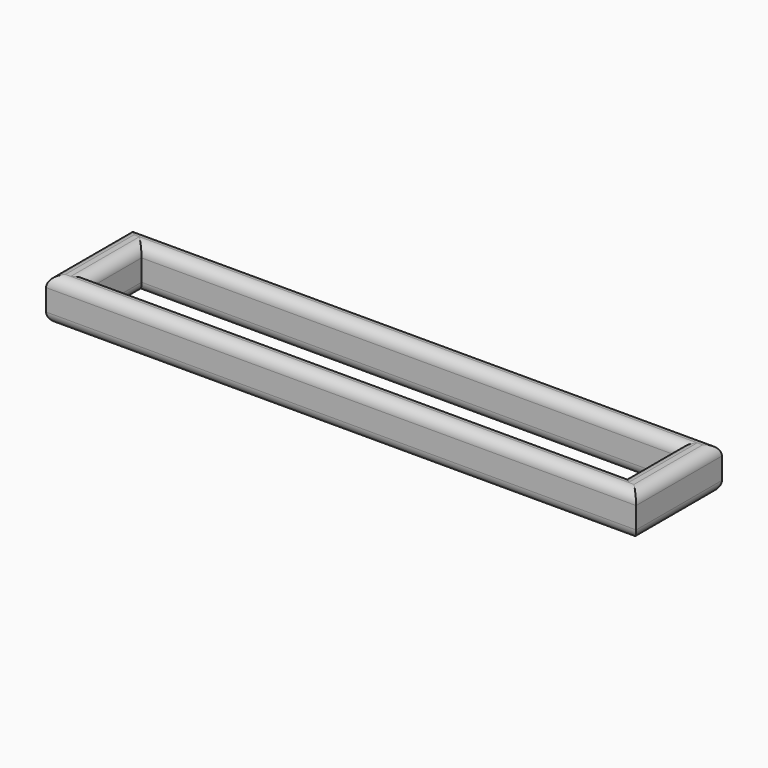
from build123d import *

# Parameters (mm, degrees)
F0_W     = 69.85
F0_H     = 12.7
F0_W_2   = 63.5
F0_H_2   = 7.62
F1_DEPTH = 5.08
F2_R     = 1.26999


# Not quite as in the source:
# - a fillet or chamfer is up to 0.001 mm smaller than in the source, because OpenCascade refuses the exact size


with BuildPart() as f1:
    # F0 (on Top) → F1 (new body)
    with BuildSketch(Plane.XY):
        Rectangle(F0_W, F0_H)
        Rectangle(F0_W_2, F0_H_2, mode=Mode.SUBTRACT)
    extrude(amount=F1_DEPTH)

    # F2 (radius 1.27 in the source; OpenCascade refuses exactly that, so slightly less here)
    f2_edges = [f1.edges().sort_by_distance(p)[0] for p in [
        (0, 6.35, 5.08),
        (-34.925, 0, 5.08),
        (0, -6.35, 5.08),
        (34.925, 0, 5.08),
        (-31.75, 0, 5.08),
        (0, 3.81, 5.08),
        (31.75, 0, 5.08),
        (0, -3.81, 5.08),
        (0, 6.35, 0),
        (-34.925, 0, 0),
        (0, -6.35, 0),
        (34.925, 0, 0),
        (-31.75, 0, 0),
        (0, 3.81, 0),
        (31.75, 0, 0),
        (0, -3.81, 0),
    ]]
    fillet(f2_edges, radius=F2_R)


solid = f1.part
